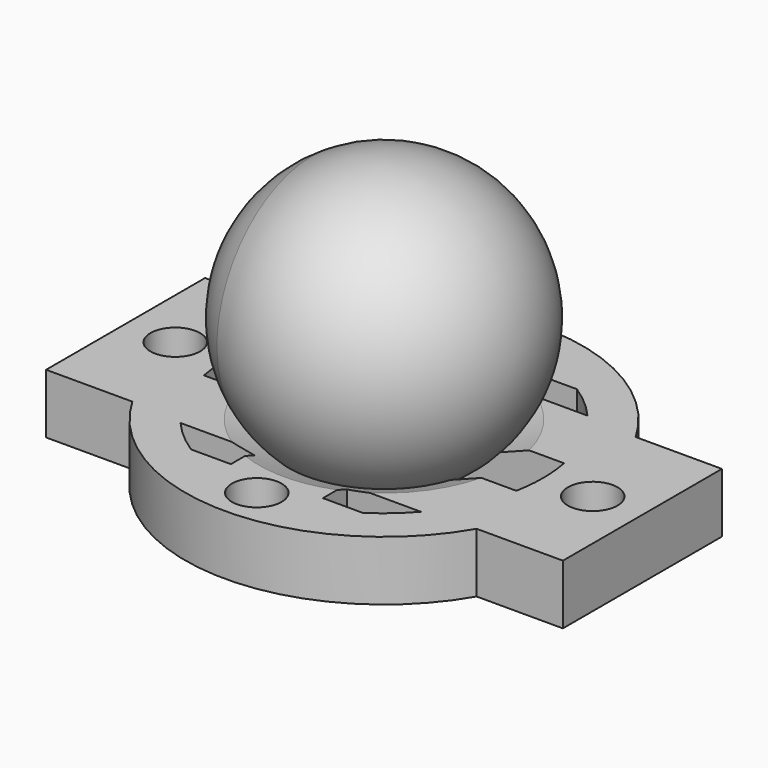
from build123d import *

# Parameters (mm, degrees)
F1_DEPTH        = 9.525
F3_DEPTH        = 9.525
F6_R            = 3.96875
F7_DEPTH        = 9.526
F7_COPIES_COUNT = 3
F7_COPIES_ANGLE = 210.7842
F9_T2_ANGLE     = 198.7595657962
F9_T4_ANGLE     = 198.7595657962


# Not quite as in the source:
# - a fillet or chamfer that OpenCascade refuses, or shapes differently, is made with other operations: its cross-section is extruded or revolved along the edge and cut away or added
# - a pattern or mirror of a feature is missing from the dataset's text; its kind, count and spacing are read off the source's solid


with BuildPart() as f1:
    # F0 (on Top) → F1 (new body)
    with BuildSketch(Plane.XY):
        with BuildLine():
            Line((-41.275, -15.875), (-27.4963065702, -15.875))
            ThreePointArc((-27.4963065702, -15.875), (0, -31.75), (27.4963065702, -15.875))
            Line((27.4963065702, -15.875), (41.275, -15.875))
            Line((41.275, -15.875), (41.275, 15.875))
            Line((41.275, 15.875), (27.4963065702, 15.875))
            ThreePointArc((27.4963065702, 15.875), (0, 31.75), (-27.4963065702, 15.875))
            Line((-27.4963065702, 15.875), (-41.275, 15.875))
            Line((-41.275, 15.875), (-41.275, -15.875))
        make_face()
    extrude(amount=F1_DEPTH)

    # F2 (on face) → F3 (cut)
    with BuildSketch(Plane.XY.offset(9.525)):
        with BuildLine():
            Line((7.3510025854, 16.625406119), (19.2030172468, 16.625406119))
            ThreePointArc((19.2030172468, 16.625406119), (16.6234467498, 19.204713436), (13.7010025854, 21.387906119))
            Line((13.7010025854, 21.387906119), (7.3510025854, 21.387906119))
            Line((7.3510025854, 21.387906119), (7.3510025854, 16.625406119))
        make_face()
        with BuildLine():
            ThreePointArc((24.9495209122, -4.7625), (25.2871294453, -2.3918788461), (25.4, 0))
            ThreePointArc((25.4, 0), (25.2871294453, 2.3918788461), (24.9495209122, 4.7625))
            Line((24.9495209122, 4.7625), (7.3510025854, 4.7625))
            Line((7.3510025854, 4.7625), (7.3510025854, -4.7625))
            Line((7.3510025854, -4.7625), (24.9495209122, -4.7625))
        make_face()
        with BuildLine():
            ThreePointArc((13.7010025854, -21.387906119), (16.6234467498, -19.204713436), (19.2030172468, -16.625406119))
            Line((19.2030172468, -16.625406119), (7.3510025854, -16.625406119))
            Line((7.3510025854, -16.625406119), (7.3510025854, -21.387906119))
            Line((7.3510025854, -21.387906119), (13.7010025854, -21.387906119))
        make_face()
    f3 = extrude(amount=-F3_DEPTH, mode=Mode.SUBTRACT)

    # F3_copies: F3 across plane
    add(f3.mirror(Plane(origin=(0, 0, 0), x_dir=(0, 0, -1), z_dir=(-1, 0, 0))), mode=Mode.SUBTRACT)

    # F4 (on Front) → F5 (revolve, cut)
    with BuildSketch(Plane.XZ):
        with BuildLine():
            Line((-22.225, 23.8125), (22.225, 23.8125))
            ThreePointArc((22.225, 23.8125), (19.3439150288, 34.7561546162), (11.4476252996, 42.8625))
            ThreePointArc((11.4476252996, 42.8625), (0, 46.0375), (-11.4476252996, 42.8625))
            ThreePointArc((-11.4476252996, 42.8625), (-19.3439150288, 34.7561546162), (-22.225, 23.8125))
        make_face()
    revolve(axis=Axis((0, 0, 23.8125), (1, 0, 0)), mode=Mode.SUBTRACT)

    # F6 (on face) → F7 (cut, through all)
    with BuildSketch(Plane.XY.offset(9.525)):
        with Locations((0, 25.4)):
            Circle(F6_R)
        with Locations((33.3375, 0)):
            Circle(F6_R)
    f7 = extrude(amount=-F7_DEPTH, mode=Mode.SUBTRACT)

    # F7_copies: F7 ×3 about axis
    f7_copies_axis = Axis((-6.99256, 0, 0), (0, 0, 1))
    for i in range(1, F7_COPIES_COUNT):
        add(f7.rotate(f7_copies_axis, i * F7_COPIES_ANGLE / (F7_COPIES_COUNT - 1)), mode=Mode.SUBTRACT)

    # F9: chamfer of 3.175 on 2 edges, made by hand

    # F9_s1 → F9_t2 (revolve, cut)
    with BuildSketch(Plane(origin=(0, 0, 0), x_dir=(0, 0, 1), z_dir=(-0.1629778352, 0.9866297306, 0))):
        with BuildLine():
            Line((9.5719539947, 20.0659493432), (7.6164291959, 15.1514665774))
            Line((7.6164291959, 15.1514665774), (7.6625695297, 15.1078395261))
            ThreePointArc((7.6625695297, 15.1078395261), (8.5706488123, 16.0878231784), (9.5658214286, 16.9754007886))
            Line((9.5658214286, 16.9754007886), (9.5885, 17.0240409054))
            ThreePointArc((9.5885, 17.0240409054), (9.5885, 18.5449951243), (9.6354539947, 20.0659493432))
            Line((9.6354539947, 20.0659493432), (9.5719539947, 20.0659493432))
        make_face()
    revolve(axis=Axis((0, 0, 9.525), (0, 0, -1)), revolution_arc=F9_T2_ANGLE, mode=Mode.SUBTRACT)

    # F9_s3 → F9_t4 (revolve, cut)
    with BuildSketch(Plane(origin=(0, 0, 0), x_dir=(0, 0, 1), z_dir=(-0.1629778352, -0.9866297306, 0))):
        with BuildLine():
            Line((9.5719539947, -20.0659493432), (7.6164291959, -15.1514665774))
            Line((7.6164291959, -15.1514665774), (7.6625695297, -15.1078395261))
            ThreePointArc((7.6625695297, -15.1078395261), (8.5706488123, -16.0878231784), (9.5658214286, -16.9754007886))
            Line((9.5658214286, -16.9754007886), (9.5885, -17.0240409054))
            ThreePointArc((9.5885, -17.0240409054), (9.5885, -18.5449951243), (9.6354539947, -20.0659493432))
            Line((9.6354539947, -20.0659493432), (9.5719539947, -20.0659493432))
        make_face()
    revolve(axis=Axis((0, 0, 9.525), (0, 0, 1)), revolution_arc=F9_T4_ANGLE, mode=Mode.SUBTRACT)


with BuildPart() as f8:
    # F4 (on Front) → F8 (revolve)
    with BuildSketch(Plane.XZ):
        with BuildLine():
            Line((-22.225, 23.8125), (22.225, 23.8125))
            ThreePointArc((22.225, 23.8125), (19.3439150288, 34.7561546162), (11.4476252996, 42.8625))
            ThreePointArc((11.4476252996, 42.8625), (0, 46.0375), (-11.4476252996, 42.8625))
            ThreePointArc((-11.4476252996, 42.8625), (-19.3439150288, 34.7561546162), (-22.225, 23.8125))
        make_face()
    revolve(axis=Axis((0, 0, 23.8125), (1, 0, 0)))


solid = Compound([f1.part, f8.part])
